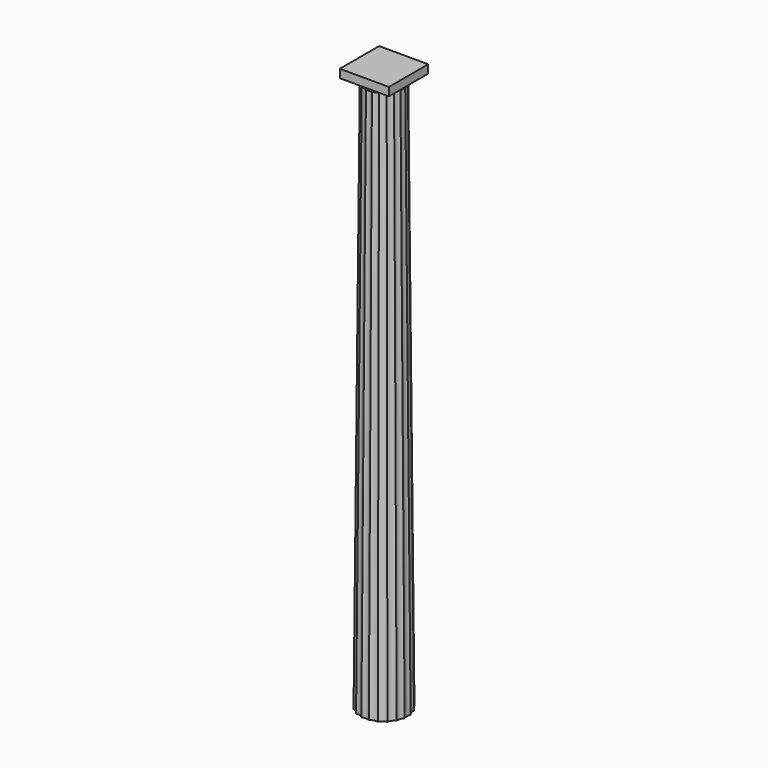
from build123d import *

# Parameters (mm, degrees)
F7_COUNT = 20
F7_ANGLE = 342
F9_DEPTH = 148
F2_R     = 125
F4_R     = 98


with BuildPart() as f6:
    # F2 (on Top) → F6 section 0
    with BuildSketch(Plane.XY):
        with BuildLine():
            Line((20.5899772422, -130), (-20.5899772422, -130))
            Line((-20.5899772422, -130), (-22.5497772005, -142.3736899553))
            ThreePointArc((-22.5497772005, -142.3736899553), (0, -137), (22.5497772005, -142.3736899553))
            Line((22.5497772005, -142.3736899553), (20.5899772422, -130))
        make_face()
    # F4 (on offset) → F6 section 1
    with BuildSketch(Plane.XY.offset(3320)):
        with BuildLine():
            Line((16.3135973534, -103), (-16.3135973534, -103))
            Line((-16.3135973534, -103), (-17.9502162781, -113.3332052143))
            ThreePointArc((-17.9502162781, -113.3332052143), (0, -110), (17.9502162781, -113.3332052143))
            Line((17.9502162781, -113.3332052143), (16.3135973534, -103))
        make_face()
    loft()


with BuildPart() as f7_1:
    # F7: instance of F6
    add(f6.part.rotate(Axis((0, 0, 1660), (0, 0, 1)), 1 * F7_ANGLE / (F7_COUNT - 1)))


with BuildPart() as f7_2:
    # F7: instance of F6
    add(f6.part.rotate(Axis((0, 0, 1660), (0, 0, 1)), 2 * F7_ANGLE / (F7_COUNT - 1)))


with BuildPart() as f7_3:
    # F7: instance of F6
    add(f6.part.rotate(Axis((0, 0, 1660), (0, 0, 1)), 3 * F7_ANGLE / (F7_COUNT - 1)))


with BuildPart() as f7_4:
    # F7: instance of F6
    add(f6.part.rotate(Axis((0, 0, 1660), (0, 0, 1)), 4 * F7_ANGLE / (F7_COUNT - 1)))


with BuildPart() as f7_5:
    # F7: instance of F6
    add(f6.part.rotate(Axis((0, 0, 1660), (0, 0, 1)), 5 * F7_ANGLE / (F7_COUNT - 1)))


with BuildPart() as f7_6:
    # F7: instance of F6
    add(f6.part.rotate(Axis((0, 0, 1660), (0, 0, 1)), 6 * F7_ANGLE / (F7_COUNT - 1)))


with BuildPart() as f7_7:
    # F7: instance of F6
    add(f6.part.rotate(Axis((0, 0, 1660), (0, 0, 1)), 7 * F7_ANGLE / (F7_COUNT - 1)))


with BuildPart() as f7_8:
    # F7: instance of F6
    add(f6.part.rotate(Axis((0, 0, 1660), (0, 0, 1)), 8 * F7_ANGLE / (F7_COUNT - 1)))


with BuildPart() as f7_9:
    # F7: instance of F6
    add(f6.part.rotate(Axis((0, 0, 1660), (0, 0, 1)), 9 * F7_ANGLE / (F7_COUNT - 1)))


with BuildPart() as f7_10:
    # F7: instance of F6
    add(f6.part.rotate(Axis((0, 0, 1660), (0, 0, 1)), 10 * F7_ANGLE / (F7_COUNT - 1)))


with BuildPart() as f7_11:
    # F7: instance of F6
    add(f6.part.rotate(Axis((0, 0, 1660), (0, 0, 1)), 11 * F7_ANGLE / (F7_COUNT - 1)))


with BuildPart() as f7_12:
    # F7: instance of F6
    add(f6.part.rotate(Axis((0, 0, 1660), (0, 0, 1)), 12 * F7_ANGLE / (F7_COUNT - 1)))


with BuildPart() as f7_13:
    # F7: instance of F6
    add(f6.part.rotate(Axis((0, 0, 1660), (0, 0, 1)), 13 * F7_ANGLE / (F7_COUNT - 1)))


with BuildPart() as f7_14:
    # F7: instance of F6
    add(f6.part.rotate(Axis((0, 0, 1660), (0, 0, 1)), 14 * F7_ANGLE / (F7_COUNT - 1)))


with BuildPart() as f7_15:
    # F7: instance of F6
    add(f6.part.rotate(Axis((0, 0, 1660), (0, 0, 1)), 15 * F7_ANGLE / (F7_COUNT - 1)))


with BuildPart() as f7_16:
    # F7: instance of F6
    add(f6.part.rotate(Axis((0, 0, 1660), (0, 0, 1)), 16 * F7_ANGLE / (F7_COUNT - 1)))


with BuildPart() as f7_17:
    # F7: instance of F6
    add(f6.part.rotate(Axis((0, 0, 1660), (0, 0, 1)), 17 * F7_ANGLE / (F7_COUNT - 1)))


with BuildPart() as f7_18:
    # F7: instance of F6
    add(f6.part.rotate(Axis((0, 0, 1660), (0, 0, 1)), 18 * F7_ANGLE / (F7_COUNT - 1)))


with BuildPart() as f7_19:
    # F7: instance of F6
    add(f6.part.rotate(Axis((0, 0, 1660), (0, 0, 1)), 19 * F7_ANGLE / (F7_COUNT - 1)))


with BuildPart() as f8:
    # F5 (on Front) → F8 (revolve)
    with BuildSketch(Plane.XZ):
        Polygon((0, 3350), (0, 3320), (118, 3320), (118, 3330), (141.8350718519, 3350), align=None)
    revolve(axis=Axis((0, 0, 3335), (0, 0, -1)))


with BuildPart() as f9:
    # F5 (on Front) → F9 (new body, symmetric)
    with BuildSketch(Plane.XZ):
        Polygon((0, 3400), (0, 3350), (141.8350718519, 3350), (143.1729889353, 3350), (148, 3350), (148, 3400), align=None)
    extrude(amount=F9_DEPTH, both=True)

    # F10: F9 across face


with BuildPart() as f9_1:
    add(f9.part)
    add(f9.part.mirror(Plane(origin=(0, 0, 3375), x_dir=(0, -1, 0), z_dir=(-1, 0, 0))))


with BuildPart() as f11:
    # F2 (on Top) → F11 section 0
    with BuildSketch(Plane.XY):
        Circle(F2_R)
    # F4 (on offset) → F11 section 1
    with BuildSketch(Plane.XY.offset(3320)):
        Circle(F4_R)
    loft()


solid = Compound([f6.part, f7_1.part, f7_2.part, f7_3.part, f7_4.part, f7_5.part, f7_6.part, f7_7.part, f7_8.part, f7_9.part, f7_10.part, f7_11.part, f7_12.part, f7_13.part, f7_14.part, f7_15.part, f7_16.part, f7_17.part, f7_18.part, f7_19.part, f8.part, f9_1.part, f11.part])
